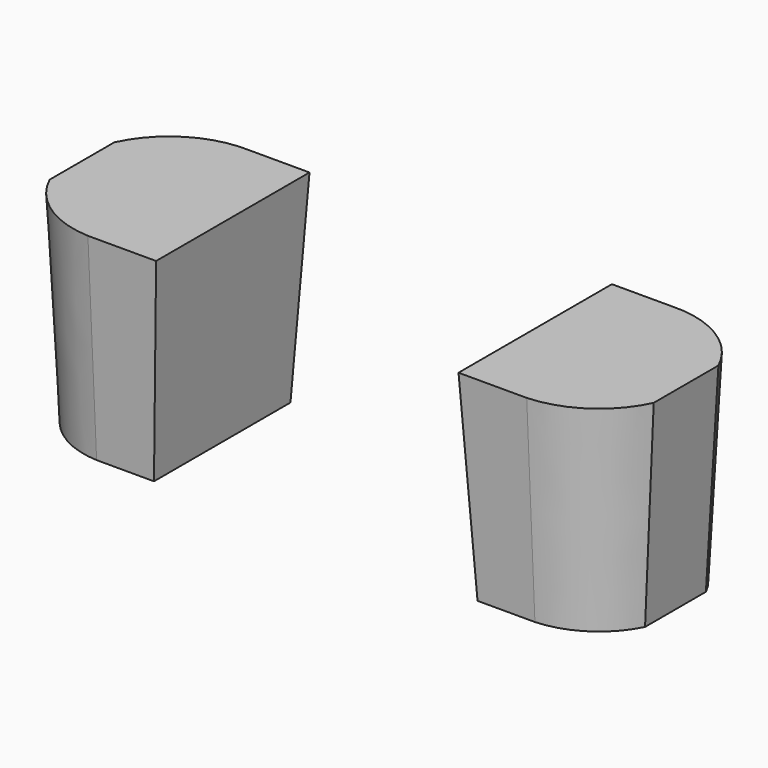
from build123d import *

# Parameters (mm, degrees)
F1_DEPTH                 = 50.8
DRAFT_F1_DRAFTED_ANGLE   = -3
DRAFT_F1_2_DRAFTED_ANGLE = -3


# Not quite as in the source:
# - an extrude with a draft is written as a straight extrude whose walls are then drafted
# - the program builds the solid bodies; features that only make, move or delete a surface that nothing else refers to are left out


with BuildPart() as f1:
    # F0 (on Top) → F1 (new body)
    with BuildSketch(Plane.XY):
        with BuildLine():
            Line((-40.7424209116, 21.3891096032), (-53.1151750277, 21.3891096032))
            ThreePointArc((-53.1151750277, 21.3891096032), (-65.0341735007, 18.4588563998), (-73.4088246416, 9.4858899614))
            Line((-73.4088246416, 9.4858899614), (-73.4088246416, -9.666296868))
            ThreePointArc((-73.4088246416, -9.666296868), (-65.9177319035, -18.0918932296), (-55.1933074071, -21.5695165098))
            Line((-55.1933074071, -21.5695165098), (-53.1151750277, -21.5695165098))
            Line((-53.1151750277, -21.5695165098), (-40.7424209116, -21.5695165098))
            Line((-40.7424209116, -21.5695165098), (-40.7424209116, 21.3891096032))
        make_face()
    extrude(amount=F1_DEPTH)

    # draft_F1_drafted
    draft_f1_drafted_walls = [f1.faces().sort_by_distance(p)[0] for p in [
        (-40.7424209116, -0.0902034533, 33.8666666667),
        (-65.9177319035, -18.0918932296, 33.8666666667),
        (-73.4088246416, -0.0902034533, 33.8666666667),
        (-65.0341735007, 18.4588563998, 33.8666666667),
        (-46.9287979697, 21.3891096032, 33.8666666667),
        (-47.9678641593, -21.5695165098, 33.8666666667),
    ]]
    draft(draft_f1_drafted_walls, neutral_plane=Plane.XY, angle=DRAFT_F1_DRAFTED_ANGLE)


with BuildPart() as f1_2:
    # F0 (on Top) → F1, piece 2 (new body)
    with BuildSketch(Plane.XY):
        with BuildLine():
            ThreePointArc((73.4088246416, 9.4858899614), (65.0341735007, 18.4588563998), (53.1151750277, 21.3891096032))
            Line((53.1151750277, 21.3891096032), (40.7424209116, 21.3891096032))
            Line((40.7424209116, 21.3891096032), (40.7424209116, -21.5695165098))
            Line((40.7424209116, -21.5695165098), (53.1151750277, -21.5695165098))
            Line((53.1151750277, -21.5695165098), (55.1933074071, -21.5695165098))
            ThreePointArc((55.1933074071, -21.5695165098), (65.9177319035, -18.0918932296), (73.4088246416, -9.666296868))
            Line((73.4088246416, -9.666296868), (73.4088246416, 9.4858899614))
        make_face()
    extrude(amount=F1_DEPTH)

    # draft_F1_2_drafted
    draft_f1_2_drafted_walls = [f1_2.faces().sort_by_distance(p)[0] for p in [
        (47.9678641593, -21.5695165098, 33.8666666667),
        (46.9287979697, 21.3891096032, 33.8666666667),
        (65.0341735007, 18.4588563998, 33.8666666667),
        (73.4088246416, -0.0902034533, 33.8666666667),
        (65.9177319035, -18.0918932296, 33.8666666667),
        (40.7424209116, -0.0902034533, 33.8666666667),
    ]]
    draft(draft_f1_2_drafted_walls, neutral_plane=Plane.XY, angle=DRAFT_F1_2_DRAFTED_ANGLE)


solid = Compound([f1.part, f1_2.part])
